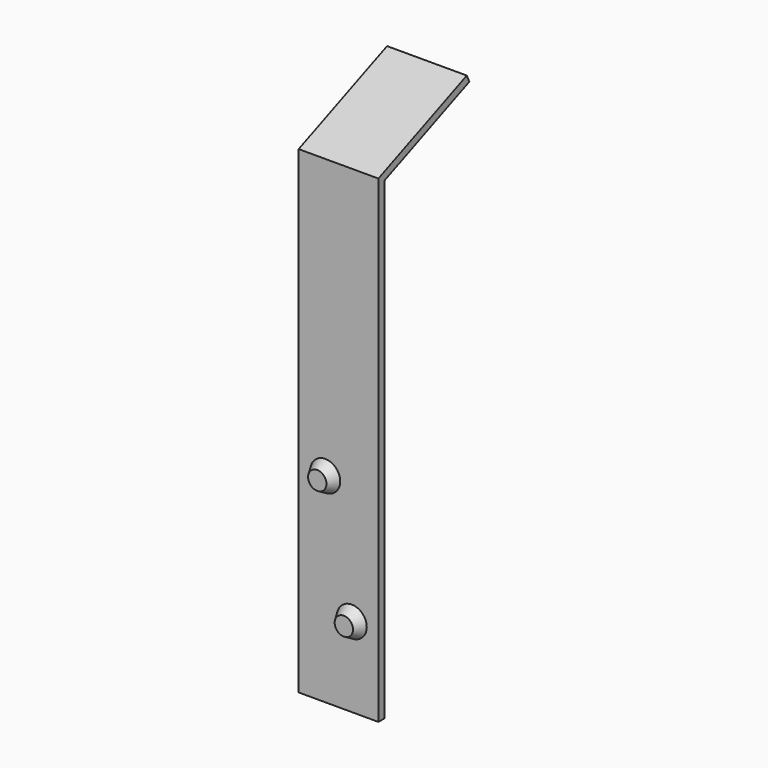
from build123d import *

# Parameters (mm, degrees)
F1_DEPTH = 50.8
F2_R     = 9.525
F3_DEPTH = 6.35
F3_TAPER = 30


# Not quite as in the source:
# - a feature names something its author has since deleted; it is built from what else it names


with BuildPart() as f1:
    # F0 (on Right) → F1 (new body)
    with BuildSketch(Plane.YZ):
        Polygon((0, 304.8), (0, 0), (4.7625, 0), (4.7625, 301.6177992369), (72.4345492237, 329.6484798189), (70.3996203774, 333.9604775462), align=None)
    extrude(amount=F1_DEPTH)

    # F2 (on face) → F3 (join)
    with BuildSketch(Plane.XZ):
        with Locations((16.9333333333, 127)):
            Circle(F2_R)
        with Locations((33.8666666667, 50.8)):
            Circle(F2_R)
    extrude(amount=F3_DEPTH, taper=F3_TAPER)


solid = f1.part
